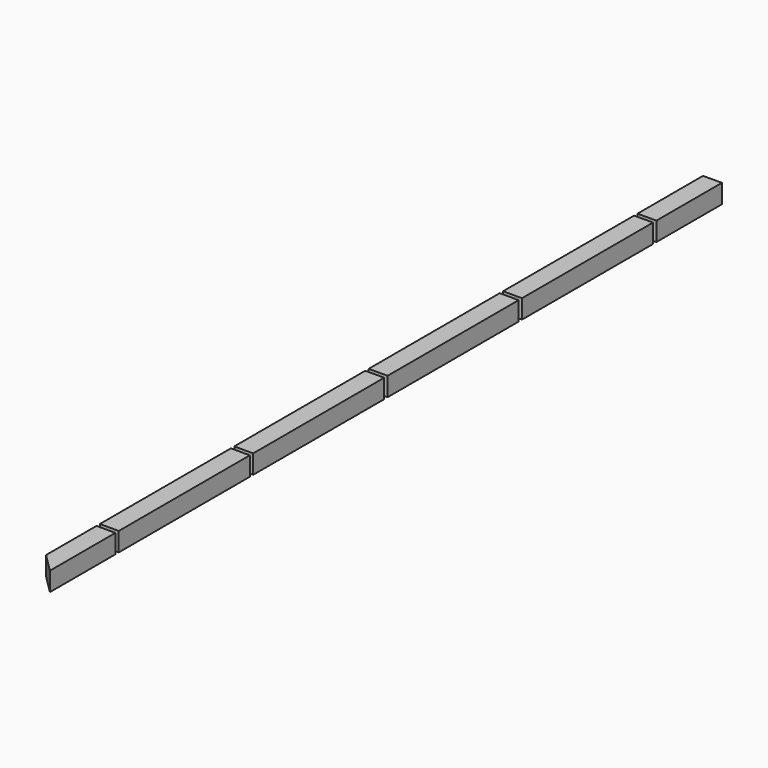
from build123d import *

# Parameters (mm, degrees)
F0_W            = 45
F0_H            = 45
F1_DEPTH        = 1500
F2_W            = 45
F2_H            = 500
F3_DEPTH        = 45
F5_DEPTH        = 5
F5_COPIES_COUNT = 3
F5_COPIES_PITCH = 400
F8_DEPTH        = 5
F11_DEPTH       = 5


# Not quite as in the source:
# - a pattern or mirror of a feature is missing from the dataset's text; its kind, count and spacing are read off the source's solid


with BuildPart() as f1:
    # F0 (on Front) → F1 (new body, symmetric)
    with BuildSketch(Plane.XZ):
        Rectangle(F0_W, F0_H)
    extrude(amount=F1_DEPTH, both=True)

    # F2 (on face) → F3 (cut, through all)
    with BuildSketch(Plane.XY.offset(22.5)):
        Polygon((22.5, -1000), (-22.5, -955), (-22.5, -1500), (22.5, -1500), align=None)
        with Locations((0, 1250)):
            Rectangle(F2_W, F2_H)
    extrude(amount=-F3_DEPTH, mode=Mode.SUBTRACT)

    # F4 (on Front) → F5 (cut, symmetric)
    with BuildSketch(Plane.XZ):
        Polygon((22.5, 22.5), (-22.5, 22.5), (-22.5, 7.5), (7.5, 7.5), (7.5, -22.5), (22.5, -22.5), align=None)
    f5 = extrude(amount=F5_DEPTH, both=True, mode=Mode.SUBTRACT)

    # F5_copies: F5 ×3
    with Locations(*[(0, i * F5_COPIES_PITCH, 0) for i in range(1, F5_COPIES_COUNT)]):
        add(f5, mode=Mode.SUBTRACT)

    # F7 (on offset) → F8 (cut, symmetric)
    with BuildSketch(Plane.XZ.offset(400)):
        Polygon((-22.5, 22.5), (-22.5, 7.5), (7.5, 7.5), (7.5, -22.5), (22.5, -22.5), (22.5, 22.5), align=None)
    extrude(amount=F8_DEPTH, both=True, mode=Mode.SUBTRACT)

    # F10 (on offset) → F11 (cut, symmetric)
    with BuildSketch(Plane.XZ.offset(800)):
        Polygon((-22.5, 22.5), (-22.5, 7.5), (7.5, 7.5), (7.5, -22.5), (22.5, -22.5), (22.5, 22.5), align=None)
    extrude(amount=F11_DEPTH, both=True, mode=Mode.SUBTRACT)


solid = f1.part
